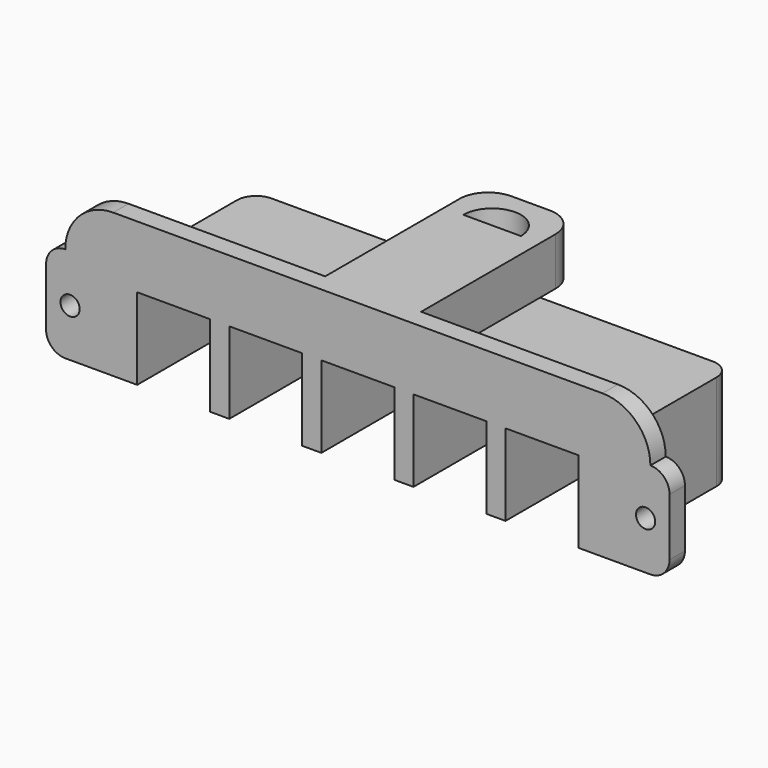
from build123d import *

# Parameters (mm, degrees)
F0_W      = 127
F0_H      = 25.4
F1_DEPTH  = 6.35
F2_W      = 19.304
F2_H      = 3.81
F3_DEPTH  = 38.1
F4_W      = 3.048
F4_H      = 5.588
F5_DEPTH  = 6.351
F6_W      = 3.048
F6_H      = 5.588
F7_DEPTH  = 6.351
F8_W      = 4.572
F8_H      = 6.858
F8_W_2    = 3.048
F8_H_2    = 5.588
F9_DEPTH  = 4.445
F10_W     = 5.08
F10_H     = 25.4
F11_DEPTH = 19.05
F12_W     = 5.08
F12_H     = 25.4
F13_DEPTH = 19.05
F14_R     = 2.54
F15_DEPTH = 5.081
F16_R     = 5.08
F17_W     = 154.94
F17_H     = 5.08
F18_DEPTH = 12.7
F19_R     = 12.69999
F20_W     = 25.4
F20_H     = 39.37
F21_DEPTH = 12.7
F22_W     = 25.4
F22_H     = 12.7
F23_DEPTH = 12.7
F25_DEPTH = 38.101
F26_R     = 7.62


# Not quite as in the source:
# - a fillet or chamfer is up to 0.001 mm smaller than in the source, because OpenCascade refuses the exact size


with BuildPart() as f1:
    # F0 (on Front) → F1 (new body)
    with BuildSketch(Plane.XZ):
        with Locations((-63.5, 12.7)):
            Rectangle(F0_W, F0_H)
    extrude(amount=F1_DEPTH)

    # F2 (on face) → F3 (join)
    with BuildSketch(Plane.XZ.offset(6.35)):
        Polygon((-121.92, 25.4), (-127, 25.4), (-127, 0), (-121.92, 0), (-121.92, 21.59), align=None)
        with Locations((-112.268, 23.495)):
            Rectangle(F2_W, F2_H)
        Polygon((-97.536, 25.4), (-102.616, 25.4), (-102.616, 21.59), (-102.616, 0), (-97.536, 0), (-97.536, 21.59), align=None)
        with Locations((-87.884, 23.495)):
            Rectangle(F2_W, F2_H)
        Polygon((-73.152, 25.4), (-78.232, 25.4), (-78.232, 21.59), (-78.232, 0), (-73.152, 0), (-73.152, 21.59), align=None)
        with Locations((-63.5, 23.495)):
            Rectangle(F2_W, F2_H)
        Polygon((-48.768, 25.4), (-53.848, 25.4), (-53.848, 21.59), (-53.848, 0), (-48.768, 0), (-48.768, 21.59), align=None)
        with Locations((-39.116, 23.495)):
            Rectangle(F2_W, F2_H)
        Polygon((-24.384, 25.4), (-29.464, 25.4), (-29.464, 21.59), (-29.464, 0), (-24.384, 0), (-24.384, 21.59), align=None)
        with Locations((-14.732, 23.495)):
            Rectangle(F2_W, F2_H)
        Polygon((0, 25.4), (-5.08, 25.4), (-5.08, 21.59), (-5.08, 0), (0, 0), align=None)
    extrude(amount=F3_DEPTH)

    # F4 (on face) → F5 (cut, through all)
    with BuildSketch(Plane.XZ.offset(6.35)):
        with Locations((-14.732, 8.636)):
            Rectangle(F4_W, F4_H)
    extrude(amount=-F5_DEPTH, mode=Mode.SUBTRACT)

    # F6 (on face) → F7 (cut, through all)
    with BuildSketch(Plane.XZ.offset(6.35)):
        with Locations((-39.116, 8.636)):
            Rectangle(F6_W, F6_H)
        with Locations((-63.5, 8.636)):
            Rectangle(F6_W, F6_H)
        with Locations((-87.884, 8.636)):
            Rectangle(F6_W, F6_H)
        with Locations((-112.268, 8.636)):
            Rectangle(F6_W, F6_H)
    extrude(amount=-F7_DEPTH, mode=Mode.SUBTRACT)

    # F8 (on face) → F9 (cut)
    with BuildSketch(Plane(origin=(0, 0, 0), x_dir=(-1, 0, 0), z_dir=(0, 1, 0))):
        with Locations((14.732, 8.636)):
            Rectangle(F8_W, F8_H)
        with Locations((14.732, 8.636)):
            Rectangle(F8_W_2, F8_H_2, mode=Mode.SUBTRACT)
        with Locations((112.268, 8.636)):
            Rectangle(F8_W, F8_H)
        with Locations((112.268, 8.636)):
            Rectangle(F8_W_2, F8_H_2, mode=Mode.SUBTRACT)
        with Locations((87.884, 8.636)):
            Rectangle(F8_W, F8_H)
        with Locations((87.884, 8.636)):
            Rectangle(F8_W_2, F8_H_2, mode=Mode.SUBTRACT)
        with Locations((63.5, 8.636)):
            Rectangle(F8_W, F8_H)
        with Locations((63.5, 8.636)):
            Rectangle(F8_W_2, F8_H_2, mode=Mode.SUBTRACT)
        with Locations((39.116, 8.636)):
            Rectangle(F8_W, F8_H)
        with Locations((39.116, 8.636)):
            Rectangle(F8_W_2, F8_H_2, mode=Mode.SUBTRACT)
    extrude(amount=-F9_DEPTH, mode=Mode.SUBTRACT)

    # F10 (on face) → F11 (join)
    with BuildSketch(Plane.YZ):
        with Locations((-41.91, 12.7)):
            Rectangle(F10_W, F10_H)
    extrude(amount=F11_DEPTH)

    # F12 (on face) → F13 (join)
    with BuildSketch(Plane(origin=(-127, 0, 0), x_dir=(0, -1, 0), z_dir=(-1, 0, 0))):
        with Locations((41.91, 12.7)):
            Rectangle(F12_W, F12_H)
    extrude(amount=F13_DEPTH)

    # F14 (on face) → F15 (cut, through all)
    with BuildSketch(Plane(origin=(0, -39.37, 0), x_dir=(-1, 0, 0), z_dir=(0, 1, 0))):
        with Locations((-12.7, 12.7)):
            Circle(F14_R)
        with Locations((139.7, 12.7)):
            Circle(F14_R)
    extrude(amount=-F15_DEPTH, mode=Mode.SUBTRACT)

    # F16
    f16_edges = [f1.edges().sort_by_distance(p)[0] for p in [
        (19.05, -41.91, 0),
        (19.05, -41.91, 25.4),
        (-146.05, -41.91, 0),
        (-146.05, -41.91, 25.4),
        (-127, 0, 12.7),
        (0, 0, 12.7),
    ]]
    fillet(f16_edges, radius=F16_R)

    # F17 (on face) → F18 (join)
    with BuildSketch(Plane.XY.offset(25.4)):
        with Locations((-63.5, -41.91)):
            Rectangle(F17_W, F17_H)
    extrude(amount=F18_DEPTH)

    # F19 (radius 12.7 in the source; OpenCascade refuses exactly that, so slightly less here)
    f19_edges = [f1.edges().sort_by_distance(p)[0] for p in [
        (13.97, -41.91, 38.1),
        (-140.97, -41.91, 38.1),
    ]]
    fillet(f19_edges, radius=F19_R)

    # F20 (on face) → F21 (join)
    with BuildSketch(Plane.XY.offset(25.4)):
        with Locations((-63.5, -19.685)):
            Rectangle(F20_W, F20_H)
    extrude(amount=F21_DEPTH)

    # F22 (on face) → F23 (join)
    with BuildSketch(Plane(origin=(0, 0, 0), x_dir=(-1, 0, 0), z_dir=(0, 1, 0))):
        with Locations((63.5, 31.75)):
            Rectangle(F22_W, F22_H)
    extrude(amount=F23_DEPTH)

    # F24 (on face) → F25 (cut, through all)
    with BuildSketch(Plane.XY.offset(38.1)):
        with BuildLine():
            ThreePointArc((-55.88, 0), (-63.5, 7.62), (-71.12, 0))
            Line((-71.12, 0), (-55.88, 0))
        make_face()
    extrude(amount=-F25_DEPTH, mode=Mode.SUBTRACT)

    # F26
    f26_edges = [f1.edges().sort_by_distance(p)[0] for p in [
        (-50.8, 12.7, 31.75),
        (-76.2, 12.7, 31.75),
    ]]
    fillet(f26_edges, radius=F26_R)


solid = f1.part
